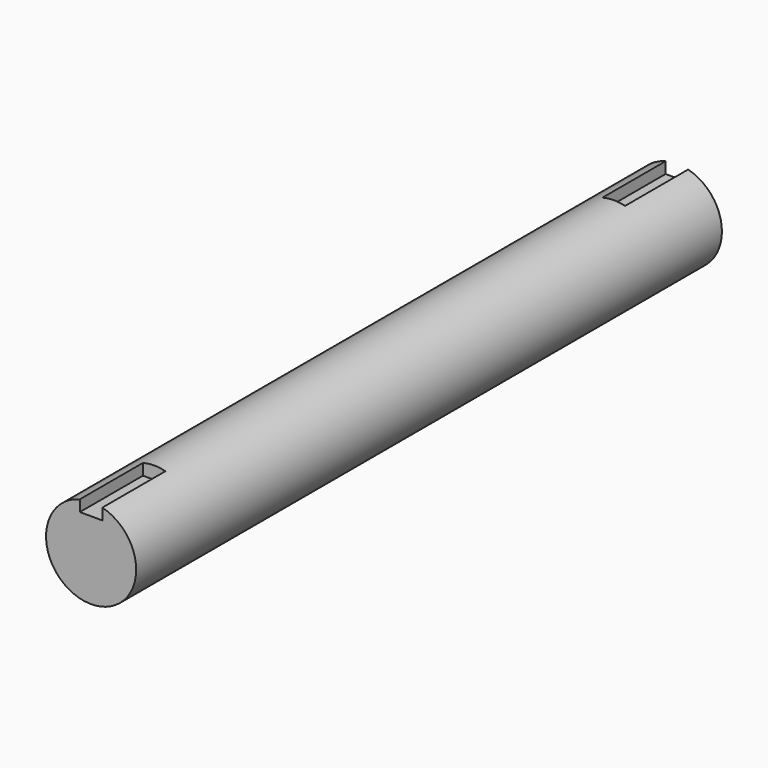
from build123d import *

# Parameters (mm, degrees)
F0_R     = 4
F1_DEPTH = 32.5
F3_DEPTH = 7


# Not quite as in the source:
# - a pattern or mirror of a feature is missing from the dataset's text; its kind, count and spacing are read off the source's solid


with BuildPart() as f1:
    # F0 (on Front) → F1 (new body, symmetric)
    with BuildSketch(Plane.XZ):
        Circle(F0_R)
    extrude(amount=F1_DEPTH, both=True)

    # F2 (on face) → F3 (cut)
    with BuildSketch(Plane.XZ.offset(32.5)):
        Polygon((0, 4.634491168), (-1, 3.8729833462), (-1, 2.8729833462), (1, 2.8729833462), (1, 3.8729833462), align=None)
    f3 = extrude(amount=-F3_DEPTH, mode=Mode.SUBTRACT)

    # F3_copies: F3 across plane
    add(f3.mirror(Plane.ZX), mode=Mode.SUBTRACT)


solid = f1.part
